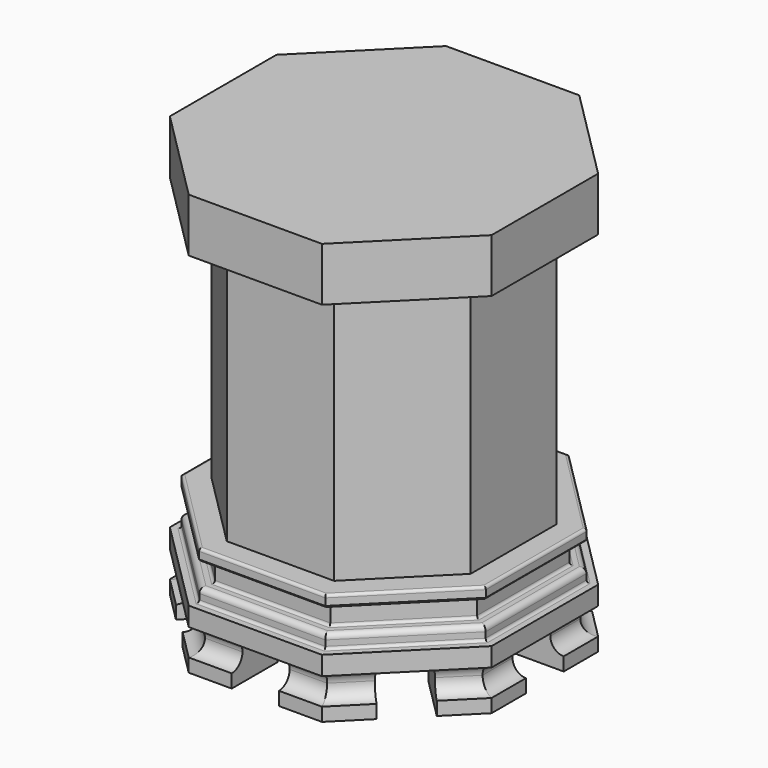
from build123d import *

# Parameters (mm, degrees)
F1_DEPTH        = 50.8
F6_DEPTH        = 123.19
F7_W            = 152.4
F7_H            = 22.3672632128
F8_DEPTH        = 19.05
F8_COPIES_COUNT = 4
F8_COPIES_ANGLE = 135
F11_DEPTH       = 19.05
F12_R           = 5.08
F14_DEPTH       = 25.4


# Not quite as in the source:
# - an extrude ends at something that could not be found from the text; its depth is read off the source's solid
# - a pattern or mirror of a feature is missing from the dataset's text; its kind, count and spacing are read off the source's solid


with BuildPart() as f1:
    # F0 (on Top) → F1 (new body)
    with BuildSketch(Plane.XY):
        Polygon((31.5630734528, 76.2), (-31.5630734528, 76.2), (-76.2, 31.5630734528), (-76.2, -31.5630734528), (-31.5630734528, -76.2), (31.5630734528, -76.2), (76.2, -31.5630734528), (76.2, 31.5630734528), align=None)
    extrude(amount=F1_DEPTH)

    # F4: sweep along a path in F2
    with BuildLine(Plane(origin=(0, 0, 0), x_dir=(1, 0, 0), z_dir=(0, 0, -1))) as f4_path:
        Line((31.5630734528, 76.2), (-31.5630734528, 76.2))
        Line((-31.5630734528, 76.2), (-76.2, 31.5630734528))
        Line((-76.2, 31.5630734528), (-76.2, -31.5630734528))
        Line((-76.2, -31.5630734528), (-31.5630734528, -76.2))
        Line((-31.5630734528, -76.2), (31.5630734528, -76.2))
        Line((31.5630734528, -76.2), (76.2, -31.5630734528))
        Line((76.2, -31.5630734528), (76.2, 31.5630734528))
        Line((76.2, 31.5630734528), (31.5630734528, 76.2))
    # F3 (on Right) → F4 (sweep, cut)
    with BuildSketch(Plane.YZ):
        with BuildLine():
            Line((-79.7076374292, 63.2637217641), (-76.2, 27.9890466481))
            Line((-76.2, 27.9890466481), (-73.3188652587, 27.9890466481))
            ThreePointArc((-73.3188652587, 27.9890466481), (-72.4208396466, 28.361021036), (-72.0488652587, 29.2590466481))
            Line((-72.0488652587, 29.2590466481), (-72.0488652587, 31.9283561945))
            ThreePointArc((-72.0488652587, 31.9283561945), (-71.3049164829, 33.7244074187), (-69.5088652587, 34.4683561945))
            Line((-69.5088652587, 34.4683561945), (-67.2529886392, 34.4683561945))
            ThreePointArc((-67.2529886392, 34.4683561945), (-66.3549630271, 34.8403305824), (-65.9829886392, 35.7383561945))
            Line((-65.9829886392, 35.7383561945), (-65.9829886392, 43.5016542661))
            ThreePointArc((-65.9829886392, 43.5016542661), (-66.3549630271, 44.3996798782), (-67.2529886392, 44.7716542661))
            Line((-67.2529886392, 44.7716542661), (-69.7752292148, 44.7716542661))
            ThreePointArc((-69.7752292148, 44.7716542661), (-70.8216576465, 44.9972239826), (-71.682225791, 45.6338688036))
            Line((-71.682225791, 45.6338688036), (-72.1423700452, 46.1568757892))
            Line((-72.1423700452, 46.1568757892), (-72.1423700452, 49.53))
            ThreePointArc((-72.1423700452, 49.53), (-71.7703956573, 50.4280256121), (-70.8723700452, 50.8))
            Line((-70.8723700452, 50.8), (-67.3975944519, 50.8))
            Line((-67.3975944519, 50.8), (-68.9155906439, 63.2637217641))
            Line((-68.9155906439, 63.2637217641), (-79.7076374292, 63.2637217641))
        make_face()
        with BuildLine():
            ThreePointArc((-76.2, 19.05), (-80.6901280605, 8.2098719395), (-69.85, 12.7))
            ThreePointArc((-69.85, 12.7), (-71.7098719395, 17.1901280605), (-76.2, 19.05))
        make_face()
    sweep(path=f4_path.line, transition=Transition.RIGHT, mode=Mode.SUBTRACT)

    # F5 (on face) → F6 (join)
    with BuildSketch(Plane.XY.offset(50.8)):
        Polygon((61.3473700452, -25.4109126886), (61.3473700452, 25.4109126886), (25.4109126886, 61.3473700452), (-25.4109126886, 61.3473700452), (-61.3473700452, 25.4109126886), (-61.3473700452, -25.4109126886), (-25.4109126886, -61.3473700452), (25.4109126886, -61.3473700452), align=None)
        Polygon((-22.7806564026, -54.997369647), (-54.997369647, -22.7806564026), (-54.997369647, 22.7806564026), (-22.7806564026, 54.997369647), (22.7806564026, 54.997369647), (54.997369647, 22.7806564026), (54.997369647, -22.7806564026), (22.7806564026, -54.997369647), align=None, mode=Mode.SUBTRACT)
    extrude(amount=F6_DEPTH)

    # F7 (on face) → F8 (cut)
    with BuildSketch(Plane(origin=(0, 0, 0), x_dir=(1, 0, 0), z_dir=(0, 0, -1))):
        Rectangle(F7_W, F7_H)
    f8 = extrude(amount=-F8_DEPTH, mode=Mode.SUBTRACT)

    # F8_copies: F8 ×4 about axis
    f8_copies_axis = Axis((0, 0, 0), (0, 0, 1))
    for i in range(1, F8_COPIES_COUNT):
        add(f8.rotate(f8_copies_axis, i * F8_COPIES_ANGLE / (F8_COPIES_COUNT - 1)), mode=Mode.SUBTRACT)

    # F10 (on face) → F11 (cut, through all)
    with BuildSketch(Plane(origin=(0, 0, 0), x_dir=(1, 0, 0), z_dir=(0, 0, -1))):
        Polygon((20.2852443943, 48.9729121327), (-20.2852443943, 48.9729121327), (-48.9729121327, 20.2852443943), (-48.9729121327, -20.2852443943), (-20.2852443943, -48.9729121327), (20.2852443943, -48.9729121327), (48.9729121327, -20.2852443943), (48.9729121327, 20.2852443943), align=None)
    extrude(amount=-F11_DEPTH, mode=Mode.SUBTRACT)

    # F12
    f12_edges = [f1.edges().sort_by_distance(p)[0] for p in [
        (62.586456, 11.183632, 19.05),
        (-62.586456, 11.183632, 19.05),
        (62.586456, -11.183632, 19.05),
        (-62.586456, -11.183632, 19.05),
        (11.183632, 62.586456, 19.05),
        (36.347286, 52.163329, 19.05),
        (-11.183632, 62.586456, 19.05),
        (52.163329, 36.347286, 19.05),
        (52.163329, -36.347286, 19.05),
        (36.347286, -52.163329, 19.05),
        (11.183632, -62.586456, 19.05),
        (-11.183632, -62.586456, 19.05),
        (-36.347286, -52.163329, 19.05),
        (-52.163329, -36.347286, 19.05),
        (-52.163329, 36.347286, 19.05),
        (-36.347286, 52.163329, 19.05),
    ]]
    fillet(f12_edges, radius=F12_R)

    # F13 (on face) → F14 (join)
    with BuildSketch(Plane.XY.offset(173.99)):
        Polygon((31.5630734528, -76.2), (76.2, -31.5630734528), (76.2, 31.5630734528), (31.5630734528, 76.2), (-31.5630734528, 76.2), (-76.2, 31.5630734528), (-76.2, -31.5630734528), (-31.5630734528, -76.2), align=None)
    extrude(amount=F14_DEPTH)


solid = f1.part
